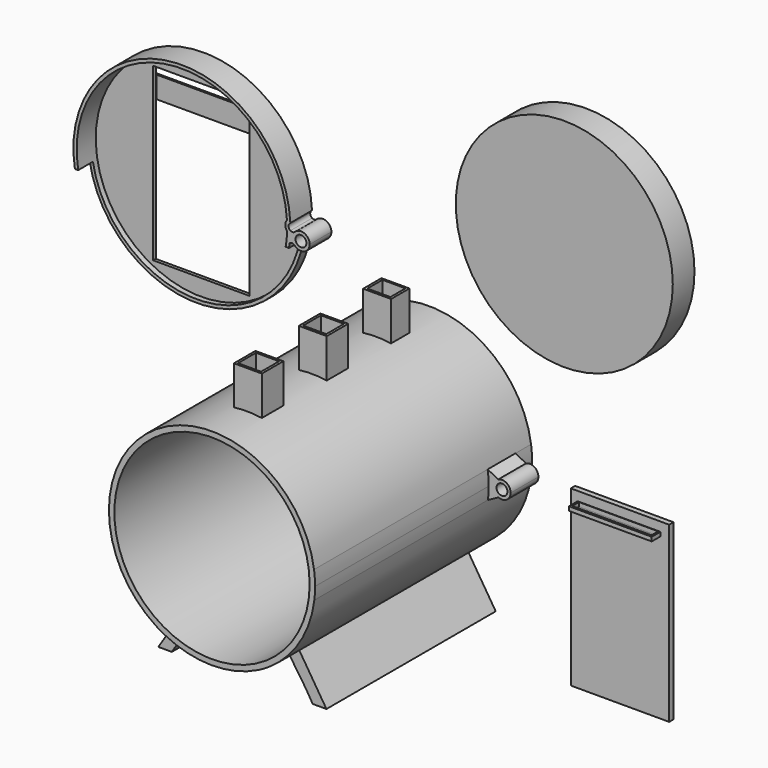
from build123d import *
from build123d import SkipClean  # not in build123d's __all__

# Parameters (mm, degrees)
F3_DEPTH  = 6.35
F0_R      = 25.4
F4_DEPTH  = 6.35
F0_R_2    = 22.86
F5_DEPTH  = 63.5
F0_R_3    = 1.27
F6_DEPTH  = 12.7
F7_T      = -0.762
F1_W      = 53.34
F1_H      = 6.3453992899
F8_DEPTH  = 25.4
F9_DEPTH  = 6.35
F10_T     = -0.762
F2_W      = 22.526679039
F2_H      = 40.0950905681
F11_DEPTH = 12.7
F12_DEPTH = 4.572
F13_DEPTH = 45.72
F14_DEPTH = 40.64
F2_W_2    = 23.0380557477
F2_H_2    = 40.64
F2_W_3    = 19.3826705217
F2_H_3    = 0.9563816711
F15_DEPTH = 1.27
F16_W     = 6.5349340439
F16_H     = 5.3656761461
F16_W_2   = 5.3930499125
F16_H_2   = 4.3982407078
F16_H_3   = 6.2861796468
F16_W_3   = 5.4061815608
F16_H_4   = 5.1973611116
F16_H_5   = 5.2650868893
F17_DEPTH = 33.02
F18_DEPTH = 22.86
F19_DEPTH = 76.8220646396
F20_DEPTH = 3.81
F21_W     = 18.5442268848
F21_H     = 1.9841159228
F22_DEPTH = 6.35
F23_DEPTH = 54.61
F24_DEPTH = 5.08


# Not quite as in the source:
# - after a boolean that leaves OpenCascade's solid faulty, fix() repairs it
# - a feature names something its author has since deleted; it is built from what else it names


with BuildPart() as f3:
    # F0 (on Front) → F3 (new body)
    with BuildSketch(Plane.XZ):
        with BuildLine():
            ThreePointArc((-32.4466640218, 29.0955113473), (-32.8887348811, 29.8733902735), (-32.4642711977, 30.661015089))
            ThreePointArc((-32.4642711977, 30.661015089), (-83.2208236821, 30.6247252425), (-32.6347884268, 26.467565851))
            ThreePointArc((-32.6347884268, 26.467565851), (-32.5066296075, 27.7790977549), (-32.4466640218, 29.0955113473))
        make_face()
    extrude(amount=-F3_DEPTH)

    # F7
    f7_openings = [f3.faces().sort_by_distance(p)[0] for p in [
        (-57.847912, 0, 29.592675),
    ]]
    offset(amount=F7_T, openings=f7_openings)

    # F1 (on Top) → F8 (cut)
    with BuildSketch(Plane.XY):
        with Locations((-57.7600412071, 1.1268389062)):
            Rectangle(F1_W, F1_H)
    extrude(amount=F8_DEPTH, mode=Mode.SUBTRACT)

    # F0 (on Front) → F9 (join)
    with BuildSketch(Plane.XZ):
        with BuildLine():
            ThreePointArc((-31.4657914959, 29.1065431926), (-31.9546424795, 28.9600756065), (-32.4466640218, 29.0955113473))
            ThreePointArc((-32.4466640218, 29.0955113473), (-32.5066296075, 27.7790977549), (-32.6347884268, 26.467565851))
            ThreePointArc((-32.6347884268, 26.467565851), (-32.1081809699, 26.6529955741), (-31.5735203503, 26.492254734))
            ThreePointArc((-31.5735203503, 26.492254734), (-31.9964212199, 27.8190453719), (-31.4657914959, 29.1065431926))
        make_face()
        with BuildLine():
            ThreePointArc((-27.9341442708, 27.7353822975), (-29.2307053411, 29.6296245156), (-31.4657914959, 29.1065431926))
            ThreePointArc((-31.4657914959, 29.1065431926), (-31.9964212199, 27.8190453719), (-31.5735203503, 26.492254734))
            ThreePointArc((-31.5735203503, 26.492254734), (-31.4295715741, 26.3677040501), (-31.3150311705, 26.2156691233))
            ThreePointArc((-31.3150311705, 26.2156691233), (-29.133051893, 25.8820120997), (-27.9341442708, 27.7353822975))
        make_face()
        with Locations((-29.9661442708, 27.7353822975)):
            Circle(F0_R_3, mode=Mode.SUBTRACT)
    extrude(amount=-F9_DEPTH)

    # F2 (on Front) → F11 (cut)
    with BuildSketch(Plane.XZ):
        with Locations((-57.7648580501, 28.8560400026)):
            Rectangle(F2_W, F2_H)
    extrude(amount=-F11_DEPTH, mode=Mode.SUBTRACT)


with BuildPart() as f4:
    # F0 (on Front) → F4 (new body)
    with BuildSketch(Plane.XZ):
        with Locations((36.7476053159, 51.4210646396)):
            Circle(F0_R)
    extrude(amount=F4_DEPTH)

    # F10
    f10_openings = [f4.faces().sort_by_distance(p)[0] for p in [
        (36.747605, 0, 51.421065),
    ]]
    offset(amount=F10_T, openings=f10_openings)


with BuildPart() as f5:
    # F0 (on Front) → F5 (new body)
    with BuildSketch(Plane.XZ):
        with BuildLine():
            ThreePointArc((23.9553467799, -2.897975268), (24.0862971189, -1.4516167195), (24.13, 0))
            ThreePointArc((24.13, 0), (24.0702094486, 1.6976210124), (23.8911340985, 3.38682912))
            ThreePointArc((23.8911340985, 3.38682912), (-12.9651224252, 20.3509827896), (-13.1661744724, -20.2214922734))
            ThreePointArc((-13.1661744724, -20.2214922734), (-12.0827697744, -20.8869235308), (-10.9658187558, -21.49436482))
            ThreePointArc((-10.9658187558, -21.49436482), (-0.1215595159, -24.1296938083), (10.7487009216, -21.6037572773))
            ThreePointArc((10.7487009216, -21.6037572773), (12.0173696309, -20.9246201197), (13.2432995784, -20.1710663148))
            ThreePointArc((13.2432995784, -20.1710663148), (20.5066999125, -12.7173959087), (23.9553467799, -2.897975268))
        make_face()
        Circle(F0_R_2, mode=Mode.SUBTRACT)
    extrude(amount=F5_DEPTH)

    # F0 (on Front) → F6 (join)
    with BuildSketch(Plane.XZ):
        with BuildLine():
            ThreePointArc((29.2741734921, 0.2885023588), (28.3358719352, 2.0010582602), (26.3875123546, 2.1320257082))
            ThreePointArc((26.3875123546, 2.1320257082), (25.2102157311, 0.2754005508), (26.4113560417, -1.5658887446))
            ThreePointArc((26.4113560417, -1.5658887446), (28.346891316, -1.4169660607), (29.2741734921, 0.2885023588))
        make_face()
        with Locations((27.2421734921, 0.2885023588)):
            Circle(F0_R_3, mode=Mode.SUBTRACT)
        with BuildLine():
            ThreePointArc((23.8911340985, 3.38682912), (24.0702094486, 1.6976210124), (24.13, 0))
            ThreePointArc((24.13, 0), (24.0862971189, -1.4516167195), (23.9553467799, -2.897975268))
            Line((23.9553467799, -2.897975268), (26.4113560417, -1.5658887446))
            ThreePointArc((26.4113560417, -1.5658887446), (25.2102157311, 0.2754005508), (26.3875123546, 2.1320257082))
            Line((26.3875123546, 2.1320257082), (23.8911340985, 3.38682912))
        make_face()
    extrude(amount=F6_DEPTH)

    # F0 (on Front) → F12 (cut)
    with BuildSketch(Plane.XZ):
        with BuildLine():
            ThreePointArc((29.2741734921, 0.2885023588), (28.3358719352, 2.0010582602), (26.3875123546, 2.1320257082))
            ThreePointArc((26.3875123546, 2.1320257082), (25.2102157311, 0.2754005508), (26.4113560417, -1.5658887446))
            ThreePointArc((26.4113560417, -1.5658887446), (28.346891316, -1.4169660607), (29.2741734921, 0.2885023588))
        make_face()
        with Locations((27.2421734921, 0.2885023588)):
            Circle(F0_R_3, mode=Mode.SUBTRACT)
        with BuildLine():
            ThreePointArc((23.8911340985, 3.38682912), (24.0702094486, 1.6976210124), (24.13, 0))
            ThreePointArc((24.13, 0), (24.0862971189, -1.4516167195), (23.9553467799, -2.897975268))
            Line((23.9553467799, -2.897975268), (26.4113560417, -1.5658887446))
            ThreePointArc((26.4113560417, -1.5658887446), (25.2102157311, 0.2754005508), (26.3875123546, 2.1320257082))
            Line((26.3875123546, 2.1320257082), (23.8911340985, 3.38682912))
        make_face()
    with SkipClean():  # cleaning this boolean's faces spoils the solid; the shape is the same uncleaned
        extrude(amount=F12_DEPTH, mode=Mode.SUBTRACT)

    # F16 (on Top) → F17 (join)
    with BuildSketch(Plane.XY):
        with Locations((0.2746605314, -12.8463576046)):
            Rectangle(F16_W, F16_H)
        with Locations((0.2654072596, -12.7893346362)):
            Rectangle(F16_W_2, F16_H_2, mode=Mode.SUBTRACT)
        with Locations((0.2746605314, -31.2107305297)):
            Rectangle(F16_W, F16_H_3)
        with Locations((0.2588414354, -31.1722606421)):
            Rectangle(F16_W_3, F16_H_4, mode=Mode.SUBTRACT)
        with Locations((0.2746605314, -50.1969101766)):
            Rectangle(F16_W, F16_H_3)
        with Locations((0.2588414354, -50.2017065883)):
            Rectangle(F16_W_3, F16_H_5, mode=Mode.SUBTRACT)
    extrude(amount=F17_DEPTH)

    add(f5.part.fix(), mode=Mode.REPLACE)

    # F16 (on Top) → F18 (cut)
    with BuildSketch(Plane.XY):
        with Locations((0.2746605314, -31.2107305297)):
            Rectangle(F16_W, F16_H_3)
        with Locations((0.2588414354, -31.1722606421)):
            Rectangle(F16_W_3, F16_H_4, mode=Mode.SUBTRACT)
        with Locations((0.2746605314, -12.8463576046)):
            Rectangle(F16_W, F16_H)
        with Locations((0.2654072596, -12.7893346362)):
            Rectangle(F16_W_2, F16_H_2, mode=Mode.SUBTRACT)
        with Locations((0.2746605314, -50.1969101766)):
            Rectangle(F16_W, F16_H_3)
        with Locations((0.2588414354, -50.2017065883)):
            Rectangle(F16_W_3, F16_H_5, mode=Mode.SUBTRACT)
    extrude(amount=F18_DEPTH, mode=Mode.SUBTRACT)

    # F16 (on Top) → F19 (cut, through all)
    with BuildSketch(Plane.XY):
        with Locations((0.2654072596, -12.7893346362)):
            Rectangle(F16_W_2, F16_H_2)
        with Locations((0.2588414354, -31.1722606421)):
            Rectangle(F16_W_3, F16_H_4)
        with Locations((0.2588414354, -50.2017065883)):
            Rectangle(F16_W_3, F16_H_5)
    extrude(amount=F19_DEPTH, mode=Mode.SUBTRACT)

    # F0 (on Front) → F23 (join)
    with BuildSketch(Plane.XZ):
        with BuildLine():
            Line((19.6842323282, -30.335681513), (13.2432995784, -20.1710663148))
            ThreePointArc((13.2432995784, -20.1710663148), (12.0173696309, -20.9246201197), (10.7487009216, -21.6037572773))
            Line((10.7487009216, -21.6037572773), (14.867214486, -27.6958085597))
            Line((14.867214486, -27.6958085597), (16.4580456913, -30.335681513))
            Line((16.4580456913, -30.335681513), (19.6842323282, -30.335681513))
        make_face()
        with BuildLine():
            ThreePointArc((-10.9658187558, -21.49436482), (-12.0827697744, -20.8869235308), (-13.1661744724, -20.2214922734))
            Line((-13.1661744724, -20.2214922734), (-19.6747548778, -30.335681513))
            Line((-19.6747548778, -30.335681513), (-16.5117273591, -30.335681513))
            Line((-16.5117273591, -30.335681513), (-14.8558095098, -27.6958085597))
            Line((-14.8558095098, -27.6958085597), (-10.9658187558, -21.49436482))
        make_face()
    extrude(amount=F23_DEPTH)

    # F0 (on Front) → F24 (cut)
    with BuildSketch(Plane.XZ):
        with BuildLine():
            Line((19.6842323282, -30.335681513), (13.2432995784, -20.1710663148))
            ThreePointArc((13.2432995784, -20.1710663148), (12.0173696309, -20.9246201197), (10.7487009216, -21.6037572773))
            Line((10.7487009216, -21.6037572773), (14.867214486, -27.6958085597))
            Line((14.867214486, -27.6958085597), (16.4580456913, -30.335681513))
            Line((16.4580456913, -30.335681513), (19.6842323282, -30.335681513))
        make_face()
        with BuildLine():
            ThreePointArc((-10.9658187558, -21.49436482), (-12.0827697744, -20.8869235308), (-13.1661744724, -20.2214922734))
            Line((-13.1661744724, -20.2214922734), (-19.6747548778, -30.335681513))
            Line((-19.6747548778, -30.335681513), (-16.5117273591, -30.335681513))
            Line((-16.5117273591, -30.335681513), (-14.8558095098, -27.6958085597))
            Line((-14.8558095098, -27.6958085597), (-10.9658187558, -21.49436482))
        make_face()
    with SkipClean():  # cleaning this boolean's faces spoils the solid; the shape is the same uncleaned
        extrude(amount=F24_DEPTH, mode=Mode.SUBTRACT)


with BuildPart() as f13:
    # F1 (on Top) → F13 (new body)
    with BuildSketch(Plane.XY):
        Polygon((-45.3702554693, 8.4333274387), (-70.1464414597, 8.4333274387), (-70.5341733992, 8.4333274387), (-70.5341733992, 6.4013274387), (-70.1464414597, 6.4013274387), (-70.1464414597, 8.0015274387), (-45.3702554693, 8.0015274387), (-45.371824471, 6.4013282079), (-44.9843034148, 6.4013274387), (-44.9843034148, 8.4333274387), align=None)
    extrude(amount=F13_DEPTH)

    # F1 (on Top) → F14 (cut)
    with BuildSketch(Plane.XY):
        Polygon((-45.3702554693, 8.4333274387), (-70.1464414597, 8.4333274387), (-70.5341733992, 8.4333274387), (-70.5341733992, 6.4013274387), (-70.1464414597, 6.4013274387), (-70.1464414597, 8.0015274387), (-45.3702554693, 8.0015274387), (-45.371824471, 6.4013282079), (-44.9843034148, 6.4013274387), (-44.9843034148, 8.4333274387), align=None)
    extrude(amount=F14_DEPTH, mode=Mode.SUBTRACT)


with BuildPart() as f15:
    # F2 (on Front) → F15 (new body)
    with BuildSketch(Plane.XZ):
        with Locations((45.7251425833, -22.1414213407)):
            Rectangle(F2_W_2, F2_H_2)
        with Locations((45.494813472, -4.4349143282)):
            Rectangle(F2_W_3, F2_H_3, mode=Mode.SUBTRACT)
    extrude(amount=F15_DEPTH)

    # F2 (on Front) → F20 (join)
    with BuildSketch(Plane.XZ):
        with Locations((45.494813472, -4.4349143282)):
            Rectangle(F2_W_3, F2_H_3)
    extrude(amount=F20_DEPTH)

    # F21 (on Top) → F22 (cut, symmetric)
    with BuildSketch(Plane.XY):
        with Locations((45.4835407436, -2.3654265096)):
            Rectangle(F21_W, F21_H)
    extrude(amount=F22_DEPTH, both=True, mode=Mode.SUBTRACT)


solid = Compound([f3.part, f4.part, f5.part, f13.part, f15.part])
